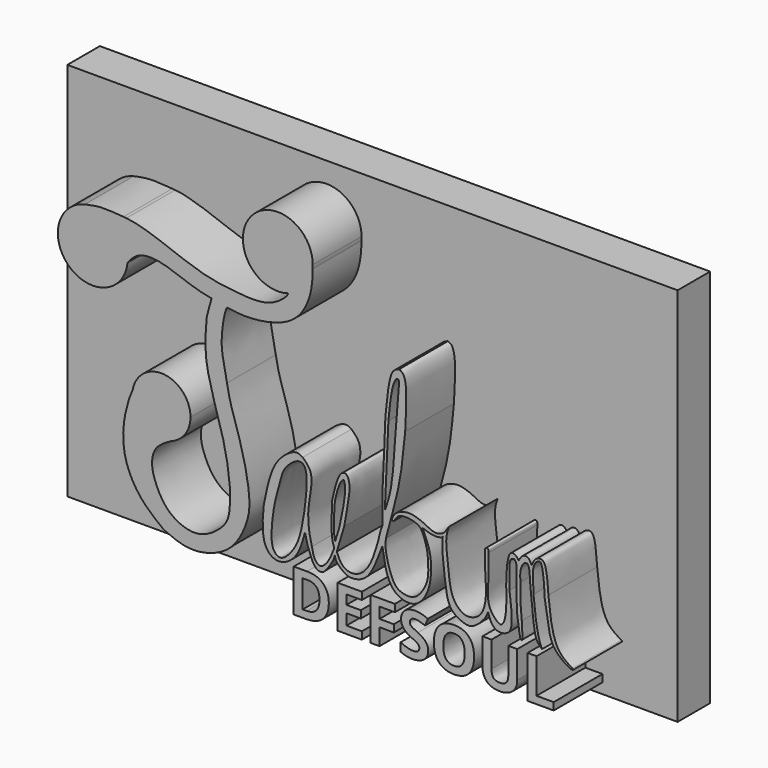
from build123d import *

# Parameters (mm, degrees)
F1_DEPTH     = 25.4
F2_W         = 152.537047863
F2_H         = 94.975899905
F3_DEPTH     = 10.16
F4_TEXT_SIZE = 14.7900181926
F5_DEPTH     = 25.4


# Not quite as in the source:
# - Text() gives the source's letters only with a copy of the font that has no kerning and outlines rounded to 1/6400 em; it was checked with that copy


with BuildPart() as f1:
    # F0 (on Front) → F1 (new body)
    with BuildSketch(Plane.XZ):
        with BuildLine():
            ThreePointArc((-48.8854791095, 27.5380207363), (-48.856621396, 27.9469284566), (-48.8469950801, 28.3567401517))
            ThreePointArc((-48.8469950801, 28.3567401517), (-50.7277701347, 33.7691105039), (-55.5595345795, 36.8489027023))
            ThreePointArc((-55.5595345795, 36.8489027023), (-57.531916112, 37.0847021636), (-59.5065325834, 36.8684151173))
            add(Edge.make_bspline(
                [(-59.6618791523, 36.831666939), (-59.6101060449, 36.8439339987), (-59.5583314354, 36.8561882455), (-59.5065325834, 36.8684151173)],
                knots=[0, 0, 0, 0, 0.0189047291, 0.0189047291, 0.0189047291, 0.0189047291], degree=3))
            ThreePointArc((-59.6618791523, 36.831666939), (-63.2752484161, 21.7471200944), (-48.8854791095, 27.5380207363))
        make_face()
        with BuildLine():
            ThreePointArc((-55.5595345795, 36.8489027023), (-50.7277701347, 33.7691105039), (-48.8469950801, 28.3567401517))
            ThreePointArc((-48.8469950801, 28.3567401517), (-48.856621396, 27.9469284566), (-48.8854791095, 27.5380207363))
            add(Edge.make_bspline(
                [(-48.8854791095, 27.5380207363), (-48.1817880442, 28.3844188674), (-46.5432478045, 30.3712369116), (-40.8942792921, 30.9688024336), (-32.8673406382, 27.4692121862), (-29.156759683, 26.7028876335), (-27.8958038306, 26.4692683239)],
                knots=[0, 0, 0, 0, 0.082166461, 0.1846550316, 0.3239505769, 0.3984097312, 0.3984097312, 0.3984097312, 0.3984097312], degree=3))
            add(Edge.make_bspline(
                [(-27.8958038306, 26.4692683239), (-27.3068098062, 26.360144458), (-26.0560871797, 26.1412987854), (-24.7541318483, 25.8804010543), (-24.0257903934, 25.7517397071)],
                knots=[0.3984097312, 0.3984097312, 0.3984097312, 0.3984097312, 0.4331896935, 0.4731389653, 0.4731389653, 0.4731389653, 0.4731389653], degree=3))
            add(Edge.make_bspline(
                [(-24.0257903934, 25.7517397071), (-22.6111441686, 25.5018427832), (-18.1577848756, 24.895804725), (-8.2092262128, 26.625170715), (-3.9292149172, 32.4283001625), (-2.7573363928, 37.0435284892), (-2.5536916805, 40.3470111453), (-2.6592031358, 41.1388377379)],
                knots=[0.4731389653, 0.4731389653, 0.4731389653, 0.4731389653, 0.5507318115, 0.6980145806, 0.8138273547, 0.9129029618, 1, 1, 1, 1], degree=3))
            ThreePointArc((-2.6592031358, 41.1388377379), (-4.6071897054, 36.5802480983), (-8.7235448528, 33.8178195511))
            add(Edge.make_bspline(
                [(-49.1537806971, 37.2068634055), (-48.6837982592, 37.1580338782), (-43.5356124304, 36.4406179167), (-31.6324676846, 31.0108603965), (-22.4662088747, 29.902672844), (-13.782298782, 29.1738320463), (-9.3082499148, 32.640941952), (-8.8616542131, 33.4745064457), (-8.7235448528, 33.8178195511)],
                knots=[0.1460032783, 0.1460032783, 0.1460032783, 0.1460032783, 0.1723906932, 0.4253166279, 0.6172365598, 0.7952587699, 0.9331574021, 1, 1, 1, 1], degree=3))
            add(Edge.make_bspline(
                [(-49.8894762828, 37.2691781432), (-49.6445798435, 37.2487754973), (-49.3991765995, 37.2278956774), (-49.1537806971, 37.2068634055)],
                knots=[0.9415582185, 0.9415582185, 0.9415582185, 0.9415582185, 1, 1, 1, 1], degree=3))
            add(Edge.make_bspline(
                [(-55.5595345795, 36.8489027023), (-54.01714731, 37.1365967988), (-52.1539060586, 37.4174241684), (-49.8894762828, 37.2691781432)],
                knots=[0, 0, 0, 0, 0.1319765562, 0.1319765562, 0.1319765562, 0.1319765562], degree=3))
        make_face()
        with BuildLine():
            ThreePointArc((-2.6006639311, 42.1480163932), (-18.3614219842, 47.317200328), (-8.7235448528, 33.8178195511))
            ThreePointArc((-8.7235448528, 33.8178195511), (-4.6071897054, 36.5802480983), (-2.6592031358, 41.1388377379))
            ThreePointArc((-2.6592031358, 41.1388377379), (-2.6153110224, 41.6425788607), (-2.6006639311, 42.1480163932))
        make_face()
        with BuildLine():
            ThreePointArc((-59.5065325834, 36.8684151173), (-57.531916112, 37.0847021636), (-55.5595345795, 36.8489027023))
            add(Edge.make_bspline(
                [(-55.5595345795, 36.8489027023), (-54.01714731, 37.1365967988), (-52.1539060586, 37.4174241684), (-49.8894762828, 37.2691781432)],
                knots=[0, 0, 0, 0, 0.1319765562, 0.1319765562, 0.1319765562, 0.1319765562], degree=3))
            add(Edge.make_bspline(
                [(-59.5065325834, 36.8684151173), (-58.3734109956, 37.1358830604), (-55.8194633618, 37.703394161), (-52.0228456872, 37.446911967), (-49.8894762828, 37.2691781432)],
                knots=[0.0189047291, 0.0189047291, 0.0189047291, 0.0189047291, 0.4324535991, 0.9415582185, 0.9415582185, 0.9415582185, 0.9415582185], degree=3))
        make_face()
        with BuildLine():
            ThreePointArc((-47.591986127, 0), (-45.2072267328, -6.857046234), (-38.0813764636, -8.2457212737))
            ThreePointArc((-38.0813764636, -8.2457212737), (-34.5127826787, -5.5903465875), (-33.1543099758, -1.3547323178))
            ThreePointArc((-33.1543099758, -1.3547323178), (-39.7563658252, 5.8958158045), (-47.591986127, 0))
        make_face()
        with BuildLine():
            add(Edge.make_bspline(
                [(-27.8958038306, 26.4692683239), (-27.3068098062, 26.360144458), (-26.0560871797, 26.1412987854), (-24.7541318483, 25.8804010543), (-24.0257903934, 25.7517397071)],
                knots=[0.3984097312, 0.3984097312, 0.3984097312, 0.3984097312, 0.4331896935, 0.4731389653, 0.4731389653, 0.4731389653, 0.4731389653], degree=3))
            add(Edge.make_bspline(
                [(-29.0722642094, 22.1029445529), (-28.7506591093, 23.2942663469), (-28.2352439627, 25.2116420338), (-27.9902828014, 26.114230582), (-27.8958038306, 26.4692683239)],
                knots=[0, 0, 0, 0, 0.6210151667, 1, 1, 1, 1], degree=3))
            add(Edge.make_bspline(
                [(-23.2720077038, -13.8276033103), (-23.5482445714, -11.2366477478), (-24.1419145271, -5.6683378867), (-27.4652636874, 4.5119283125), (-29.82113025, 13.5844870668), (-29.3171383854, 19.3174660503), (-29.0722642094, 22.1029445529)],
                knots=[0, 0, 0, 0, 0.2358023573, 0.5067707878, 0.7603550665, 1, 1, 1, 1], degree=3))
            add(Edge.make_bspline(
                [(-38.0813764636, -8.2457212737), (-39.4965978279, -9.0581706762), (-42.2162009703, -10.6118314872), (-43.0718107283, -14.9187147421), (-41.8754342745, -19.0076930727), (-38.9499231045, -24.5491342692), (-31.6078794094, -27.6441519413), (-25.9614434698, -23.9701917502), (-23.1820488908, -20.6600770338), (-23.2396353932, -16.2863040672), (-23.2720077038, -13.8276033103)],
                knots=[0, 0, 0, 0, 0.1167079371, 0.224030729, 0.3353525523, 0.4696995112, 0.6152186582, 0.7497687049, 0.8593382239, 1, 1, 1, 1], degree=3))
            ThreePointArc((-38.0813764636, -8.2457212737), (-45.2072267328, -6.857046234), (-47.591986127, 0))
            add(Edge.make_bspline(
                [(-47.591986127, 0), (-47.9959058789, -0.9730347754), (-48.9554577917, -3.2845765494), (-50.3109203944, -9.7820981866), (-49.577496568, -16.8906195541), (-45.6394948892, -23.7857354453), (-41.7471919223, -26.8214810182), (-39.8227795959, -28.3223986626)],
                knots=[0, 0, 0, 0, 0.1476042441, 0.3506486971, 0.5638765084, 0.7843740761, 1, 1, 1, 1], degree=3))
            add(Edge.make_bspline(
                [(-39.8227795959, -28.3223986626), (-37.8892989971, -29.1659474385), (-34.0033354432, -30.8613354352), (-27.3951575392, -29.855922843), (-21.8542680853, -26.3992098193), (-18.8661274411, -19.935248928), (-18.0415356918, -15.0297783192), (-19.8557518031, -4.699324068), (-23.1249044009, 4.262724528), (-23.7642356239, 7.7036287655), (-24.0257903934, 9.1113261878)],
                knots=[0, 0, 0, 0, 0.1196386605, 0.2404531364, 0.3614295677, 0.4853454063, 0.5917684837, 0.7464093139, 0.8962543185, 1, 1, 1, 1], degree=3))
            add(Edge.make_bspline(
                [(-24.0257903934, 9.1113261878), (-24.3226990401, 10.6432025909), (-24.9039099446, 13.6419137423), (-25.6557543679, 17.4684052369), (-24.8217541558, 23.9196136729), (-24.233894145, 25.2727325976), (-24.0257903934, 25.7517397071)],
                knots=[0, 0, 0, 0, 0.2638234694, 0.5164453074, 0.8288205631, 1, 1, 1, 1], degree=3))
        make_face()
    extrude(amount=F1_DEPTH)



with BuildPart() as f1b:
    # F0 (on Front) → F1, piece 2 (new body)
    with BuildSketch(Plane.XZ):
        with BuildLine():
            add(Edge.make_bspline(
                [(-5.1085525192, -1.0792703833), (-4.3672149582, -1.8017652254), (-2.7778664515, -3.3334580925), (-2.8892315083, -7.4567305526), (-4.1642077766, -13.3362448616), (-3.4048535221, -17.7289134169), (-2.8061070479, -19.9905186892)],
                knots=[0, 0, 0, 0, 0.1985569306, 0.4217517623, 0.7018450077, 1, 1, 1, 1], degree=3))
            add(Edge.make_bspline(
                [(-5.1085525192, -1.0792703833), (-5.478783997, -0.8527364186), (-6.2897286764, -0.3565427547), (-8.2247993049, -0.8681471283), (-11.2606205616, -3.3933698947), (-12.9970998351, -6.8182780711), (-13.6686487673, -9.4381761324), (-14.0083450824, -10.76342538)],
                knots=[0, 0, 0, 0, 0.1341236027, 0.2937805901, 0.5271693526, 0.7608233431, 1, 1, 1, 1], degree=3))
            add(Edge.make_bspline(
                [(-14.0083450824, -10.76342538), (-14.3506180106, -12.1821005673), (-15.0650098837, -15.1431586613), (-15.2083138365, -20.4421358162), (-14.4776735687, -24.4080639034), (-11.2990956592, -26.5950853985), (-7.2123704696, -24.5193654879), (-5.4381393642, -20.772287153), (-4.826056849, -18.5002745533), (-4.5329411514, -17.4122471362)],
                knots=[0, 0, 0, 0, 0.1508635661, 0.3148823546, 0.4548811843, 0.581449398, 0.7239636206, 0.8678109669, 1, 1, 1, 1], degree=3))
            add(Edge.make_bspline(
                [(-4.5329411514, -17.4122471362), (-4.3131276252, -18.4117032653), (-3.8888098592, -20.3410067039), (-2.834426151, -22.7858974951), (-2.1012479524, -24.3252222931), (-0.3771592902, -25.1662751983), (0.904032805, -23.9011937371), (2.6455407022, -21.286750405), (2.8523203824, -20.3534698985), (2.9327366501, -19.9905186892)],
                knots=[0, 0, 0, 0, 0.1728632961, 0.3336872344, 0.4623956914, 0.5853407919, 0.7114282933, 0.8877749517, 1, 1, 1, 1], degree=3))
            add(Edge.make_bspline(
                [(2.9327366501, -19.9905186892), (3.0098366233, -20.447673615), (3.2020361206, -21.4799049623), (5.2472622659, -23.1478983948), (6.4021652157, -23.6760882029), (8.6145357084, -23.7020609064), (11.7457098955, -22.0792086855), (13.8081754778, -16.687584113), (14.5253828175, -14.8803824509), (14.8178655654, -14.1402501613)],
                knots=[0, 0, 0, 0, 0.1079048248, 0.2491952521, 0.3504694348, 0.4766379043, 0.640208577, 0.8524965928, 1, 1, 1, 1], degree=3))
            add(Edge.make_bspline(
                [(14.8178655654, -14.1402501613), (15.03599069, -15.6726231911), (15.4564115272, -18.6261644365), (16.8586822499, -22.4588760323), (19.6482233252, -24.5874716103), (23.764879924, -24.6418914179), (26.7589811027, -20.0472726922), (27.1650299593, -14.5510257359), (26.5636040431, -10.6130706212), (25.4109934707, -8.1180548454), (24.8297769576, -6.8599157967)],
                knots=[0, 0, 0, 0, 0.1306176902, 0.2517564118, 0.3619405594, 0.4765157987, 0.6127482211, 0.7559198045, 0.8769198865, 1, 1, 1, 1], degree=3))
            add(Edge.make_bspline(
                [(24.8297769576, -6.8599157967), (25.2260052605, -7.0008175456), (26.0581793908, -7.2967448923), (27.5651527881, -7.7067966982), (28.8442226506, -7.6542125758), (29.3809674694, -7.4985245942), (29.616959393, -7.4300728738)],
                knots=[0, 0, 0, 0, 0.2591850494, 0.5443505462, 0.7996634763, 1, 1, 1, 1], degree=3))
            Line((29.616959393, -7.4300728738), (29.904525727, -7.1348054335))
            add(Edge.make_bspline(
                [(29.904525727, -7.1348054335), (29.8709061299, -7.458989189), (29.7928985427, -8.211193105), (29.7799963671, -10.0857686429), (29.8657140324, -10.9575265659), (29.904525727, -11.3522456959)],
                knots=[0, 0, 0, 0, 0.2930174633, 0.6798887347, 1, 1, 1, 1], degree=3))
            add(Edge.make_bspline(
                [(29.904525727, -11.3522456959), (30.0517713826, -12.7501744548), (30.3700341478, -15.7717146866), (31.0943697999, -22.1930971018), (34.0259866174, -24.0895004), (36.8972189713, -25.0744651414), (38.4285278607, -23.7764286014), (39.2037406564, -23.1193080544)],
                knots=[0, 0, 0, 0, 0.2193514264, 0.4741151189, 0.6589723256, 0.8273574857, 1, 1, 1, 1], degree=3))
            add(Edge.make_bspline(
                [(39.2037406564, -23.1193080544), (39.7554980251, -22.5164533766), (40.7466364279, -21.4335273362), (41.0654923175, -20.4341061422), (41.206844151, -19.9910532683)],
                knots=[0, 0, 0, 0, 0.556690536, 1, 1, 1, 1], degree=3))
            add(Edge.make_bspline(
                [(41.206844151, -19.9910532683), (41.4455207588, -20.7836642789), (41.9071421845, -22.316643267), (43.6454246209, -23.8865988217), (46.7952549926, -23.223668734), (47.367990589, -19.738372467), (46.8733860244, -15.8560365845), (46.5797781944, -13.5513991117)],
                knots=[0, 0, 0, 0, 0.1747725865, 0.3380254617, 0.5182358851, 0.7140145351, 1, 1, 1, 1], degree=3))
            add(Edge.make_bspline(
                [(46.5797781944, -13.5513991117), (46.5888672818, -12.2268924122), (46.6056045951, -9.7878484487), (46.5095078203, -6.5543627845), (47.4088371677, -6.3431190588), (47.7420762181, -6.2648444436)],
                knots=[0, 0, 0, 0, 0.4279316633, 0.78802481, 1, 1, 1, 1], degree=3))
            add(Edge.make_bspline(
                [(47.7420762181, -6.2648444436), (47.9408881014, -6.4920250408), (48.542703509, -7.1797142343), (48.1715606399, -11.627837644), (48.3531732925, -15.6098582395), (48.4543591738, -17.8284496069)],
                knots=[0, 0, 0, 0, 0.1792973476, 0.5427437463, 1, 1, 1, 1], degree=3))
            add(Edge.make_bspline(
                [(48.4543591738, -17.8284496069), (48.7311618564, -19.7946043892), (49.1140224241, -22.5140980339), (49.2872524916, -23.3941328124), (49.6239712336, -23.5608858827), (49.9970375024, -23.1603164539), (49.7002282084, -21.8887532239), (49.6992448176, -19.9101573227), (49.6617020312, -19.4035166048), (49.6480949223, -19.2198883742)],
                knots=[0, 0, 0, 0, 0.2931979374, 0.40553772, 0.4721219743, 0.553838251, 0.7043648089, 0.8928491826, 1, 1, 1, 1], degree=3))
            add(Edge.make_bspline(
                [(49.2749176919, -10.86808553), (49.2479568791, -12.1025971642), (49.1913652027, -14.6938796813), (49.4911371707, -17.6644998857), (49.6480949223, -19.2198883742)],
                knots=[0, 0, 0, 0, 0.47640951, 1, 1, 1, 1], degree=3))
            add(Edge.make_bspline(
                [(49.2749176919, -10.86808553), (49.2414512202, -9.8969162516), (49.1804134755, -8.1256514788), (50.079492076, -6.1953837577), (51.5539698838, -6.0507378962), (51.6581828306, -9.5743673921), (51.855411038, -11.5187169118), (51.9551075995, -12.5015629455)],
                knots=[0, 0, 0, 0, 0.2238917084, 0.4083443586, 0.5307098991, 0.7627793204, 1, 1, 1, 1], degree=3))
            add(Edge.make_bspline(
                [(51.9551075995, -12.5015629455), (52.142068565, -14.3637146778), (52.4924720557, -17.8537718961), (53.0170238252, -22.2924203759), (54.2129821712, -23.3978364599), (54.7068119049, -23.8542798907)],
                knots=[0, 0, 0, 0, 0.4017573704, 0.7529763478, 1, 1, 1, 1], degree=3))
            add(Edge.make_bspline(
                [(52.5846853852, -12.5015629455), (52.7123677662, -13.883884298), (52.9761071027, -16.7391922376), (53.7658812013, -21.6754594265), (54.4357217964, -23.2265432531), (54.7068119049, -23.8542798907)],
                knots=[0, 0, 0, 0, 0.3584192418, 0.7403468846, 1, 1, 1, 1], degree=3))
            add(Edge.make_bspline(
                [(52.5846853852, -12.5015629455), (52.5852023104, -12.3955191168), (52.5869484806, -12.0373037201), (52.5599873391, -9.587958848), (52.2499774519, -7.6242939874), (52.8962920676, -5.2121922987), (53.8971662236, -4.7985080651), (54.7053546122, -4.6699783373), (55.299693318, -9.5819655086), (55.3621058226, -11.5822488859), (55.3907901049, -12.5015629455)],
                knots=[0, 0, 0, 0, 0.0598503696, 0.2021741778, 0.3417568913, 0.4824675167, 0.5734679812, 0.636423713, 0.8329032795, 1, 1, 1, 1], degree=3))
            add(Edge.make_bspline(
                [(55.3907901049, -12.5015629455), (55.6977147496, -14.5456145837), (56.274326594, -18.3857245434), (57.2733831929, -22.898028164), (61.143839339, -25.6547428709), (61.9468163306, -25.8731013161), (62.2068978846, -25.943826884)],
                knots=[0, 0, 0, 0, 0.3184168583, 0.5982019858, 0.869858971, 1, 1, 1, 1], degree=3))
            add(Edge.make_bspline(
                [(62.2068978846, -25.943826884), (62.2768708564, -25.9599040096), (62.4196275792, -25.9927040709), (62.5978405511, -25.7339803345), (62.4347302793, -25.6350016251), (62.3507983983, -25.584070012)],
                knots=[0, 0, 0, 0, 0.3181890434, 0.6491595811, 1, 1, 1, 1], degree=3))
            add(Edge.make_bspline(
                [(56.3081689179, -11.4402789623), (56.4345292534, -12.780207198), (56.6979437255, -15.5734610102), (57.6035303854, -20.4254376498), (59.045461805, -23.1701966893), (60.7520051351, -24.6512491972), (61.8331120618, -25.2820243371), (62.3507983983, -25.584070012)],
                knots=[0, 0, 0, 0, 0.2317695964, 0.4831537177, 0.6806345947, 0.8470723824, 1, 1, 1, 1], degree=3))
            add(Edge.make_bspline(
                [(52.1001927555, -6.2648444436), (52.2966671486, -5.7772902037), (52.6748391302, -4.838850593), (53.8206407313, -4.0050509893), (55.3783116106, -4.1683022991), (56.0462045771, -7.5020473709), (56.2162798605, -10.0588680889), (56.3081689179, -11.4402789623)],
                knots=[0, 0, 0, 0, 0.1710072668, 0.3291531069, 0.4779354199, 0.7179365442, 1, 1, 1, 1], degree=3))
            add(Edge.make_bspline(
                [(48.8613806665, -6.2648444436), (49.1513298189, -5.7241400653), (49.6915133173, -4.7167924657), (51.381104018, -4.5432847135), (51.8486544362, -5.662640267), (52.1001927555, -6.2648444436)],
                knots=[0, 0, 0, 0, 0.3486757794, 0.6495928709, 1, 1, 1, 1], degree=3))
            add(Edge.make_bspline(
                [(46.223051846, -6.8326233886), (46.3599384202, -6.1871717537), (46.6083920444, -5.0156558547), (48.1511233355, -5.1143053387), (48.6184368093, -5.8713019967), (48.8613806665, -6.2648444436)],
                knots=[0, 0, 0, 0, 0.3707084832, 0.6728480625, 1, 1, 1, 1], degree=3))
            add(Edge.make_bspline(
                [(45.7657426596, -12.3117435724), (45.8123268532, -10.86808553), (45.8887775935, -8.4988543078), (46.129147855, -7.3006993234), (46.223051846, -6.8326233886)],
                knots=[0, 0, 0, 0, 0.6093360702, 1, 1, 1, 1], degree=3))
            add(Edge.make_bspline(
                [(41.3306728005, -7.0211407728), (41.3681649082, -8.5189877674), (41.4477431077, -11.6982159984), (40.8585286931, -17.8753135037), (42.4562761896, -20.4941468821), (44.5461265435, -22.4396820417), (45.9121285753, -19.5808077515), (45.8238287402, -15.1961156496), (45.7657426596, -12.3117435724)],
                knots=[0, 0, 0, 0, 0.1815123852, 0.3852658525, 0.5314469786, 0.6501921464, 0.7698866918, 1, 1, 1, 1], degree=3))
            add(Edge.make_bspline(
                [(40.4367595911, -6.7049786448), (40.4504729984, -6.5476909599), (40.477104051, -6.2422426855), (40.8887845034, -6.0504646683), (41.3762497952, -6.2140582542), (41.3474165536, -6.7246405216), (41.3306728005, -7.0211407728)],
                knots=[0, 0, 0, 0, 0.2375580928, 0.4613311557, 0.6871895914, 1, 1, 1, 1], degree=3))
            add(Edge.make_bspline(
                [(31.4524173737, -4.4802846387), (31.1665474901, -5.2691332258), (30.4511658942, -7.2432053252), (31.3000578143, -13.3212821079), (31.8195905902, -19.5407650072), (34.2314111827, -22.119608782), (36.0438719697, -22.921625642), (39.3341012166, -22.0543029015), (41.0198597051, -17.7442989446), (40.4373171028, -11.3519474502), (40.4369348872, -8.1661055724), (40.4367595911, -6.7049786448)],
                knots=[0, 0, 0, 0, 0.090573042, 0.2266565703, 0.3646972754, 0.4621600057, 0.5361988242, 0.6293867971, 0.7425565045, 0.8819283448, 1, 1, 1, 1], degree=3))
            add(Edge.make_bspline(
                [(30.7932887226, -5.3710956126), (31.012998273, -5.0741586213), (31.2327078233, -4.77722163), (31.4524173737, -4.4802846387)],
                knots=[0, 0, 0, 0, 1.1081492543, 1.1081492543, 1.1081492543, 1.1081492543], degree=3))
            add(Edge.make_bspline(
                [(17.3738077283, -6.9408607669), (17.5954154741, -6.537182398), (18.0907045801, -5.6349689047), (20.23637222, -4.7671344907), (22.3712456999, -4.6210908521), (25.3012125491, -5.7130688126), (26.7133499072, -6.6074980573), (28.6389259321, -7.1277805896), (30.4527421277, -6.1728889636), (30.6968306118, -5.5981995481), (30.7932887226, -5.3710956126)],
                knots=[0, 0, 0, 0, 0.1098174977, 0.2454400232, 0.3823598081, 0.5426984774, 0.6636963571, 0.7903620221, 0.9171559307, 1, 1, 1, 1], degree=3))
            add(Edge.make_bspline(
                [(17.8145114332, -7.5434544124), (17.7704731381, -7.6102261849), (17.6722143493, -7.7592081895), (17.2354082712, -7.729331386), (17.1137986341, -7.3756887109), (17.2799069848, -7.097896302), (17.3738077283, -6.9408607669)],
                knots=[0, 0, 0, 0, 0.2085102063, 0.4652305514, 0.6976958195, 1, 1, 1, 1], degree=3))
            add(Edge.make_bspline(
                [(15.6817473471, -12.1709787086), (15.603301068, -12.9589602384), (15.407716217, -14.9235817824), (17.1738425615, -20.984074886), (19.0841660956, -22.8883614829), (23.1804845275, -23.48613861), (25.7560252839, -19.4080611405), (26.3472668389, -16.9542252287), (26.2686825498, -13.4707346788), (26.0055149918, -11.00449224), (24.8715315439, -7.6637380655), (23.6940769046, -6.2395230906), (20.1432221876, -5.6201467501), (18.4223552545, -6.3875679754), (18.0039759544, -7.1831653667), (17.8145114332, -7.5434544124)],
                knots=[0, 0, 0, 0, 0.074583997, 0.1859552816, 0.2591434544, 0.3427739221, 0.4362540989, 0.5095607023, 0.5912928701, 0.6645519847, 0.7469893196, 0.8074641837, 0.8903710072, 0.9503541293, 1, 1, 1, 1], degree=3))
            add(Edge.make_bspline(
                [(20.5076914281, 12.8999240696), (20.1944413152, 9.7037216227), (19.6197822773, 3.8402708278), (18.3460840842, -2.3631812073), (16.6376760145, -8.6520711077), (15.6817473471, -12.1709787086)],
                knots=[0, 0, 0, 0, 0.3454663783, 0.6337599524, 1, 1, 1, 1], degree=3))
            add(Edge.make_bspline(
                [(18.9950987697, 26.1199828237), (19.3307966721, 25.9794090083), (20.2503562664, 25.594342555), (20.9813160465, 21.9593726972), (20.6459058392, 16.3577755884), (20.5494943793, 13.9457513267), (20.5076914281, 12.8999240696)],
                knots=[0, 0, 0, 0, 0.1481967021, 0.4059474258, 0.7424253213, 1, 1, 1, 1], degree=3))
            add(Edge.make_bspline(
                [(15.6817473471, 15.7653130591), (15.7954931504, 16.8686916013), (16.0492771822, 19.3304954402), (16.8319575461, 25.3455723906), (18.4124974784, 25.9114099791), (18.9950987697, 26.1199828237)],
                knots=[0, 0, 0, 0, 0.3389942735, 0.7563473204, 1, 1, 1, 1], degree=3))
            add(Edge.make_bspline(
                [(14.8178655654, -2.311981516), (14.9794651671, 0.5910102342), (15.2866861511, 6.1099593716), (15.4517673748, 13.4468342352), (15.6216256818, 15.159213291), (15.6817473471, 15.7653130591)],
                knots=[0, 0, 0, 0, 0.4175668963, 0.7938467141, 1, 1, 1, 1], degree=3))
            add(Edge.make_bspline(
                [(14.4245913252, -10.631035082), (14.5840973229, -10.3076422474), (14.9761174558, -9.5128351311), (14.7501613509, -6.9714378784), (14.7928557596, -4.0331756795), (14.8178655654, -2.311981516)],
                knots=[0, 0, 0, 0, 0.2212764816, 0.5438343197, 1, 1, 1, 1], degree=3))
            add(Edge.make_bspline(
                [(3.412916325, -19.071303308), (3.8059536161, -20.0464545632), (4.5714049838, -21.9455895279), (7.5596252958, -22.9923696681), (11.0912260349, -21.1038778754), (13.3058635912, -15.3993080808), (14.0632911974, -12.1709787086), (14.4245913252, -10.631035082)],
                knots=[0, 0, 0, 0, 0.1742063231, 0.3392717976, 0.5292552706, 0.7754503144, 1, 1, 1, 1], degree=3))
            add(Edge.make_bspline(
                [(3.412916325, -19.071303308), (3.7571241134, -18.0300083016), (4.436686443, -15.9691315548), (4.9879717455, -13.9410636933), (5.2582793869, -12.9377152771)],
                knots=[0, 0, 0, 0, 0.505373576, 1, 1, 1, 1], degree=3))
            add(Edge.make_bspline(
                [(2.2049085237, -9.6600623801), (2.1736096189, -9.361569239), (2.0761947533, -8.4325421698), (3.2818017925, -3.5497791985), (4.4689612183, -1.2508531356), (5.9308892504, -0.9388419974), (6.7546711179, -3.25611473), (6.4494611325, -6.0883015242), (5.6659474293, -10.7849528145), (5.3768196881, -12.3201663333), (5.2582793869, -12.9377152771)],
                knots=[0, 0, 0, 0, 0.0838172177, 0.2608786783, 0.3872436642, 0.4648117539, 0.5756071461, 0.7136111699, 0.8847620143, 1, 1, 1, 1], degree=3))
            add(Edge.make_bspline(
                [(2.7805198915, -18.5002745533), (2.6202349761, -18.0503977209), (2.24744619, -17.004079433), (2.0720636818, -14.4225922527), (2.112646697, -11.1160611515), (2.1788695269, -10.0709879888), (2.2049085237, -9.6600623801)],
                knots=[0, 0, 0, 0, 0.2092610076, 0.48669681, 0.7981677903, 1, 1, 1, 1], degree=3))
            add(Edge.make_bspline(
                [(2.5182997342, -19.1390812397), (2.6057064533, -18.9261456776), (2.6931131724, -18.7132101155), (2.7805198915, -18.5002745533)],
                knots=[0, 0, 0, 0, 0.69053124, 0.69053124, 0.69053124, 0.69053124], degree=3))
            add(Edge.make_bspline(
                [(-2.8061070479, -19.9905186892), (-2.6225181003, -20.9371406268), (-2.2982275572, -22.6092485949), (-0.6806116711, -24.0092619653), (1.3025122933, -22.2127615599), (2.082810635, -20.2400584573), (2.5182997342, -19.1390812397)],
                knots=[0, 0, 0, 0, 0.2643852132, 0.4670086378, 0.7025343823, 1, 1, 1, 1], degree=3))
        make_face()
        with BuildLine():
            add(Edge.make_bspline(
                [(-4.8926980235, -2.6622016449), (-5.2013683457, -2.3473382356), (-6.3600942602, -1.8804956938), (-9.8626150799, -4.6930654549), (-10.8049578054, -8.3070282539), (-12.341615005, -13.7241956374), (-13.2008746282, -21.3342468848), (-12.3951094669, -24.2831823398), (-10.390235379, -25.5923442915), (-7.1304058883, -22.2093557381), (-5.2788854617, -17.5230361985), (-4.111256501, -8.9647171712), (-4.0181384442, -4.4338450424), (-4.543807061, -3.0180926716), (-4.8926980235, -2.6622016449)],
                knots=[0, 0, 0, 0, 0.0483951518, 0.1319473589, 0.2126597334, 0.313091932, 0.4290683798, 0.4994929505, 0.5534930822, 0.6361996846, 0.7330679023, 0.8564266507, 0.9452988193, 1, 1, 1, 1], degree=3))
        make_face(mode=Mode.SUBTRACT)
        with BuildLine():
            add(Edge.make_bspline(
                [(3.0263895169, -16.8507769704), (3.3399987133, -15.9778852224), (4.0939342696, -13.8794004427), (5.1955942673, -8.0155989048), (5.6903627187, -4.2975223514), (5.3129485602, -3.1413720799), (5.1655182615, -2.6897420175)],
                knots=[0, 0, 0, 0, 0.2377278958, 0.5715123006, 0.8326187078, 1, 1, 1, 1], degree=3))
            add(Edge.make_bspline(
                [(3.0263895169, -16.8507769704), (2.8832174548, -16.2452530024), (2.5538045092, -14.8520521847), (2.7654806196, -11.3455482199), (2.7794974126, -7.9281751943), (4.1513554615, -3.3432836175), (4.9170082221, -2.849885585), (5.1655182615, -2.6897420175)],
                knots=[0, 0, 0, 0, 0.1692826724, 0.3894887241, 0.6222573856, 0.8773950323, 1, 1, 1, 1], degree=3))
        make_face(mode=Mode.SUBTRACT)
        with BuildLine():
            add(Edge.make_bspline(
                [(15.4177583754, -6.2648444436), (16.0002471697, -4.5534862401), (17.3864704312, -0.4807477196), (17.9630039486, 11.0398837407), (18.3818214195, 15.7291437623), (18.5639504343, 17.7683383226)],
                knots=[0, 0, 0, 0, 0.2905633763, 0.6914909181, 1, 1, 1, 1], degree=3))
            add(Edge.make_bspline(
                [(16.3160320371, 13.9072462916), (16.0166074832, 7.1832160465), (15.7171829293, 0.4591858014), (15.4177583754, -6.2648444436)],
                knots=[0, 0, 0, 0, 20.1920811261, 20.1920811261, 20.1920811261, 20.1920811261], degree=3))
            add(Edge.make_bspline(
                [(18.5639504343, 17.7683383226), (18.6822912649, 19.4051530607), (18.8677704209, 21.9705822083), (19.0672920737, 23.5195422417), (18.4874788143, 24.1265006524), (17.4401650429, 22.5573531278), (16.7242465116, 18.3168176107), (16.4527485085, 15.3840705316), (16.3160320371, 13.9072462916)],
                knots=[0, 0, 0, 0, 0.2235723521, 0.3504116961, 0.4228408574, 0.5484461336, 0.7726139767, 1, 1, 1, 1], degree=3))
        make_face(mode=Mode.SUBTRACT)
    extrude(amount=F1_DEPTH)


with BuildPart() as f1_1:
    add(f1.part)

    add(f1b.part)  # F3 merges F1b
    # F2 (on Front) → F3 (join)
    with BuildSketch(Plane.XZ):
        with Locations((0.1439005136, 8.4902700037)):
            Rectangle(F2_W, F2_H)
    extrude(amount=F3_DEPTH)

    # F4 (on Front) → F5 (join)
    with BuildSketch(Plane.XZ):
        with Locations((-8.6718581151, -36.4074297249)):
            Text('DEFSOUL', F4_TEXT_SIZE, font='Open Sans', font_style=FontStyle.BOLD, text_align=(TextAlign.LEFT, TextAlign.BOTTOM))
    extrude(amount=F5_DEPTH)


solid = f1_1.part
